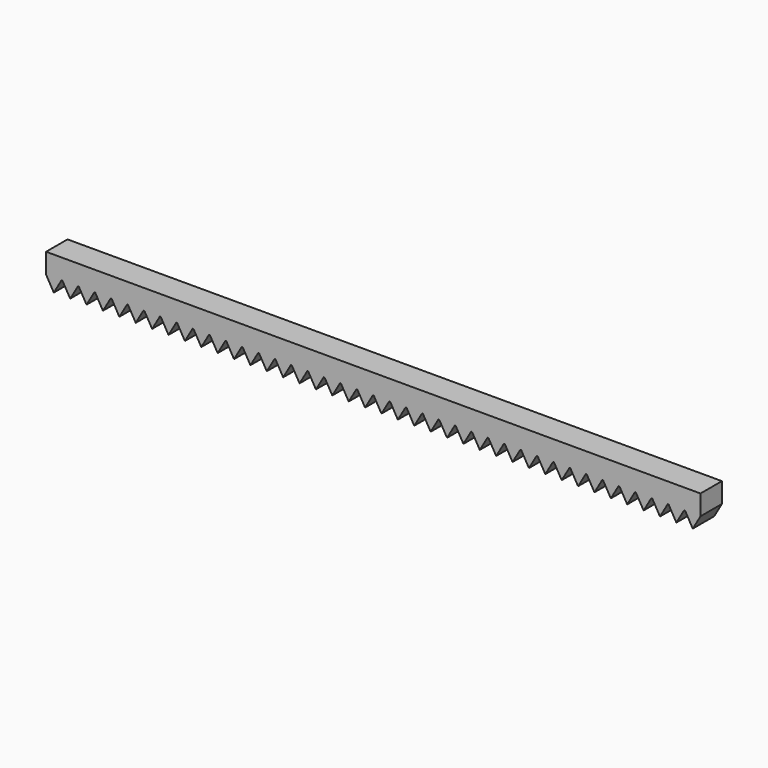
from build123d import *

# Parameters (mm, degrees)
F1_DEPTH = 4


# Not quite as in the source:
# - ends of sketch curves that miss each other by under 0.0002 mm in the source are joined


with BuildPart() as f1:
    # F0 (on Front) → F1 (new body)
    with BuildSketch(Plane.XZ):
        Polygon((48.878435, 1.5), (-48.878435, 1.5), (-48.878435, -1.5), (-46.5690339232, -1.5), (-46.4310674122, -1.5), (-44.1216663354, -1.5), (-43.9836963354, -1.5), (-41.6742952587, -1.5), (-41.5363252587, -1.5), (-39.22692239, -1.5), (-39.08895239, -1.5), (-36.7795513132, -1.5), (-36.6415813132, -1.5), (-34.3321802365, -1.5), (-34.1942102365, -1.5), (-31.8848091597, -1.5), (-31.7468391597, -1.5), (-29.4374380829, -1.5), (-29.2994680829, -1.5), (-26.9900670062, -1.5), (-26.8520970062, -1.5), (-24.5426959294, -1.5), (-24.4047259294, -1.5), (-22.0953248527, -1.5), (-21.9573548527, -1.5), (-19.6479537759, -1.5), (-19.5099837759, -1.5), (-17.2005822649, -1.5), (-17.062612265, -1.5), (-14.7532111882, -1.5), (-14.6152411882, -1.5), (-12.3058401114, -1.5), (-12.1678701114, -1.5), (-9.8584690347, -1.5), (-9.7204990347, -1.5), (-7.4110979579, -1.5), (-7.2731279579, -1.5), (-4.9637268812, -1.5), (-4.8257568812, -1.5), (-2.5163558044, -1.5), (-2.3783858044, -1.5), (-0.0689847276, -1.5), (0.0689852724, -1.5), (2.3783863491, -1.5), (2.5163563491, -1.5), (4.8257574259, -1.5), (4.9637274259, -1.5), (7.2731285026, -1.5), (7.4110985026, -1.5), (9.7204995794, -1.5), (9.8584695794, -1.5), (12.1678706561, -1.5), (12.3058406561, -1.5), (14.6152417329, -1.5), (14.7532117329, -1.5), (17.0626128097, -1.5), (17.2005828097, -1.5), (19.5099838864, -1.5), (19.6479538864, -1.5), (21.5619457761, -1.5), (21.9573549632, -1.5), (22.0953249632, -1.5), (23.8713468528, -1.5), (24.4047260399, -1.5), (24.5426960399, -1.5), (26.8520971167, -1.5), (26.9900671167, -1.5), (29.2994681935, -1.5), (29.4374381935, -1.5), (31.7468392702, -1.5), (31.8848092702, -1.5), (34.194210347, -1.5), (34.332180347, -1.5), (36.6415814237, -1.5), (36.7795514237, -1.5), (39.0889525005, -1.5), (39.2269225005, -1.5), (41.5363235773, -1.5), (41.6742935773, -1.5), (43.983694654, -1.5), (44.121664654, -1.5), (46.4310657308, -1.5), (46.5690357308, -1.5), (48.878435, -1.5), align=None)
        Polygon((-46.5690339232, -1.5), (-48.878435, -1.5), (-47.7237344616, -3.5), align=None)
        Polygon((47.7237362691, -3.5), (48.8784368075, -1.5), (46.5690357308, -1.5), align=None)
        Polygon((-44.1216663354, -1.5), (-46.4310674122, -1.5), (-45.2763668738, -3.5), align=None)
        Polygon((45.2763651924, -3.5), (46.4310657308, -1.5), (44.121664654, -1.5), align=None)
        Polygon((-41.6742952587, -1.5), (-43.9836963354, -1.5), (-42.8289957971, -3.5), align=None)
        Polygon((42.8289941156, -3.5), (43.983694654, -1.5), (41.6742935773, -1.5), align=None)
        Polygon((-39.22692239, -1.5), (-41.5363252587, -1.5), (-40.3816238243, -3.5), align=None)
        Polygon((40.3816230389, -3.5), (41.5363235773, -1.5), (39.2269225005, -1.5), align=None)
        Polygon((-36.7795513132, -1.5), (-39.08895239, -1.5), (-37.9342518516, -3.5), align=None)
        Polygon((37.9342519621, -3.5), (39.0889525005, -1.5), (36.7795514237, -1.5), align=None)
        Polygon((-34.3321802365, -1.5), (-36.6415813132, -1.5), (-35.4868807748, -3.5), align=None)
        Polygon((35.4868808854, -3.5), (36.6415814237, -1.5), (34.332180347, -1.5), align=None)
        Polygon((-31.8848091597, -1.5), (-34.1942102365, -1.5), (-33.0395096981, -3.5), align=None)
        Polygon((33.0395098086, -3.5), (34.194210347, -1.5), (31.8848092702, -1.5), align=None)
        Polygon((-29.4374380829, -1.5), (-31.7468391597, -1.5), (-30.5921386213, -3.5), align=None)
        Polygon((30.5921387318, -3.5), (31.7468392702, -1.5), (29.4374381935, -1.5), align=None)
        Polygon((-26.9900670062, -1.5), (-29.2994680829, -1.5), (-28.1447675446, -3.5), align=None)
        Polygon((28.1447676551, -3.5), (29.2994681935, -1.5), (26.9900671167, -1.5), align=None)
        Polygon((-24.5426959294, -1.5), (-26.8520970062, -1.5), (-25.6973964678, -3.5), align=None)
        Polygon((25.6973965783, -3.5), (26.8520971167, -1.5), (24.5426960399, -1.5), align=None)
        Polygon((-22.0953248527, -1.5), (-24.4047259294, -1.5), (-23.250025391, -3.5), align=None)
        Polygon((23.2500255016, -3.5), (24.4047260399, -1.5), (23.8713468528, -1.5), (22.0953249632, -1.5), align=None)
        Polygon((-19.6479537759, -1.5), (-21.9573548527, -1.5), (-20.8026543143, -3.5), align=None)
        Polygon((20.8026544248, -3.5), (21.9573549632, -1.5), (21.5619457761, -1.5), (19.6479538864, -1.5), align=None)
        Polygon((-17.2005822649, -1.5), (-19.5099837759, -1.5), (-18.3552830204, -3.500000376), align=None)
        Polygon((-14.7532111882, -1.5), (-17.062612265, -1.5), (-15.9079117266, -3.5), align=None)
        Polygon((18.355283348, -3.5), (19.5099838864, -1.5), (17.2005828097, -1.5), align=None)
        Polygon((-12.3058401114, -1.5), (-14.6152411882, -1.5), (-13.4605406498, -3.5), align=None)
        Polygon((15.9079122713, -3.5), (17.0626128097, -1.5), (14.7532117329, -1.5), align=None)
        Polygon((-9.8584690347, -1.5), (-12.1678701114, -1.5), (-11.0131695731, -3.5), align=None)
        Polygon((13.4605411945, -3.5), (14.6152417329, -1.5), (12.3058406561, -1.5), align=None)
        Polygon((-7.4110979579, -1.5), (-9.7204990347, -1.5), (-8.5657984963, -3.5), align=None)
        Polygon((11.0131701178, -3.5), (12.1678706561, -1.5), (9.8584695794, -1.5), align=None)
        Polygon((-4.9637268812, -1.5), (-7.2731279579, -1.5), (-6.1184274195, -3.5), align=None)
        Polygon((8.565799041, -3.5), (9.7204995794, -1.5), (7.4110985026, -1.5), align=None)
        Polygon((-2.5163558044, -1.5), (-4.8257568812, -1.5), (-3.6710563428, -3.5), align=None)
        Polygon((6.1184279642, -3.5), (7.2731285026, -1.5), (4.9637274259, -1.5), align=None)
        Polygon((-0.0689847276, -1.5), (-2.3783858044, -1.5), (-1.223685266, -3.5), align=None)
        Polygon((3.6710568875, -3.5), (4.8257574259, -1.5), (2.5163563491, -1.5), align=None)
        Polygon((2.3783863491, -1.5), (0.0689852724, -1.5), (1.2236858107, -3.5), align=None)
    extrude(amount=F1_DEPTH)


solid = f1.part
